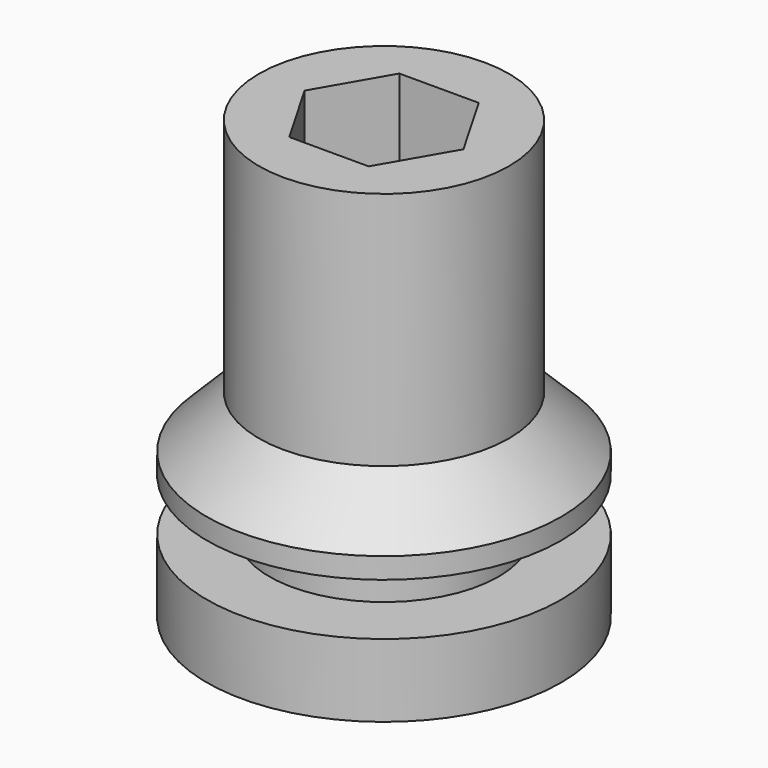
from build123d import *

# Parameters (mm, degrees)
F0_R        = 8.5
F1_DEPTH    = 11
F3_DEPTH    = 2
F5_R        = 8.5
F5_R_2      = 5.5
F6_DEPTH    = 2.5
F7_R        = 6
F8_DEPTH    = 10
F9_S5_R     = 6
F9_T6_DEPTH = 14
F11_DEPTH   = 12


# Not quite as in the source:
# - a fillet or chamfer that OpenCascade refuses, or shapes differently, is made with other operations: its cross-section is extruded or revolved along the edge and cut away or added


with BuildPart() as f1:
    # F0 (on Top) → F1 (new body)
    with BuildSketch(Plane.XY):
        Circle(F0_R)
    extrude(amount=F1_DEPTH)

    # F2 (on face) → F3 (cut)
    with BuildSketch(Plane(origin=(0, 0, 0), x_dir=(1, 0, 0), z_dir=(0, 0, -1))):
        Polygon((7, 4.0414518843), (0, 8.0829037687), (-7, 4.0414518843), (-7, -4.0414518843), (0, -8.0829037687), (7, -4.0414518843), align=None)
    extrude(amount=-F3_DEPTH, mode=Mode.SUBTRACT)

    # F5 (on offset) → F6 (cut)
    with BuildSketch(Plane(origin=(0, 0, 3.5), x_dir=(1, 0, 0), z_dir=(0, 0, -1))):
        Circle(F5_R)
        Circle(F5_R_2, mode=Mode.SUBTRACT)
    extrude(amount=-F6_DEPTH, mode=Mode.SUBTRACT)

    # F7 (on face) → F8 (join)
    with BuildSketch(Plane.XY.offset(11)):
        Circle(F7_R)
    extrude(amount=F8_DEPTH)

    # F9: chamfer of 4 on 1 edges, made by hand


with BuildPart() as f9_tool2:
    # F9_s3 → F9_t4 (revolve)
    with BuildSketch(Plane.XZ):
        Polygon((8.5, 7), (4.5, 11), (8.5, 11), align=None)
    revolve(axis=Axis((0, 0, 11), (0, 0, 1)))

    # F9_s5 → F9_t6 (cut, symmetric)
    with BuildSketch(Plane.XY.offset(9)):
        Circle(F9_S5_R)
    extrude(amount=F9_T6_DEPTH, both=True, mode=Mode.SUBTRACT)


with BuildPart() as f1_1:
    add(f1.part)

    # F9_t1: cut F9_tool2
    add(f9_tool2.part, mode=Mode.SUBTRACT)

    # F10 (on face) → F11 (cut)
    with BuildSketch(Plane.XY.offset(21)):
        Polygon((3.8105117767, 0), (1.9052558883, 3.3), (-1.9052558883, 3.3), (-3.8105117767, 0), (-1.9052558883, -3.3), (1.9052558883, -3.3), align=None)
    extrude(amount=-F11_DEPTH, mode=Mode.SUBTRACT)


solid = f1_1.part
